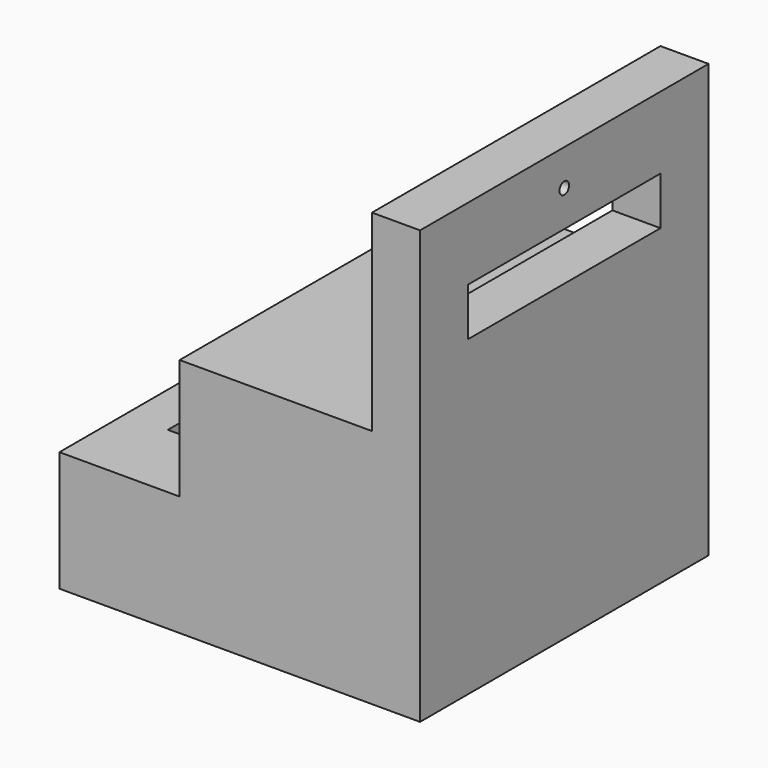
from build123d import *

# Parameters (mm, degrees)
F1_DEPTH = 150
F2_W     = 100
F2_H     = 20
F3_DEPTH = 20.001
F4_R     = 2.5
F5_DEPTH = 20.001
F6_W     = 20
F6_H     = 80
F7_DEPTH = 25.4
F8_W     = 20
F8_H     = 80
F9_DEPTH = 75.401


with BuildPart() as f1:
    # F0 (on Front) → F1 (new body)
    with BuildSketch(Plane.XZ):
        Polygon((75, -90), (75, 90), (55, 90), (55, 10), (-25, 10), (-25, -40), (-75, -40), (-75, -90), align=None)
    extrude(amount=F1_DEPTH)

    # F2 (on face) → F3 (cut, through all)
    with BuildSketch(Plane(origin=(55, 0, 0), x_dir=(0, -1, 0), z_dir=(-1, 0, 0))):
        with Locations((75, 50)):
            Rectangle(F2_W, F2_H)
    extrude(amount=-F3_DEPTH, mode=Mode.SUBTRACT)

    # F4 (on face) → F5 (cut, through all)
    with BuildSketch(Plane(origin=(55, 0, 0), x_dir=(0, -1, 0), z_dir=(-1, 0, 0))):
        with Locations((75, 75)):
            Circle(F4_R)
    extrude(amount=-F5_DEPTH, mode=Mode.SUBTRACT)

    # F6 (on face) → F7 (join)
    with BuildSketch(Plane.XY.offset(-40)):
        with Locations((-47.3200663872, -75.7392449304)):
            Rectangle(F6_W, F6_H)
    extrude(amount=F7_DEPTH)

    # F8 (on face) → F9 (cut, through all)
    with BuildSketch(Plane.XY.offset(-14.6)):
        with Locations((-47.3200663872, -75.7392449304)):
            Rectangle(F8_W, F8_H)
    extrude(amount=-F9_DEPTH, mode=Mode.SUBTRACT)


solid = f1.part
